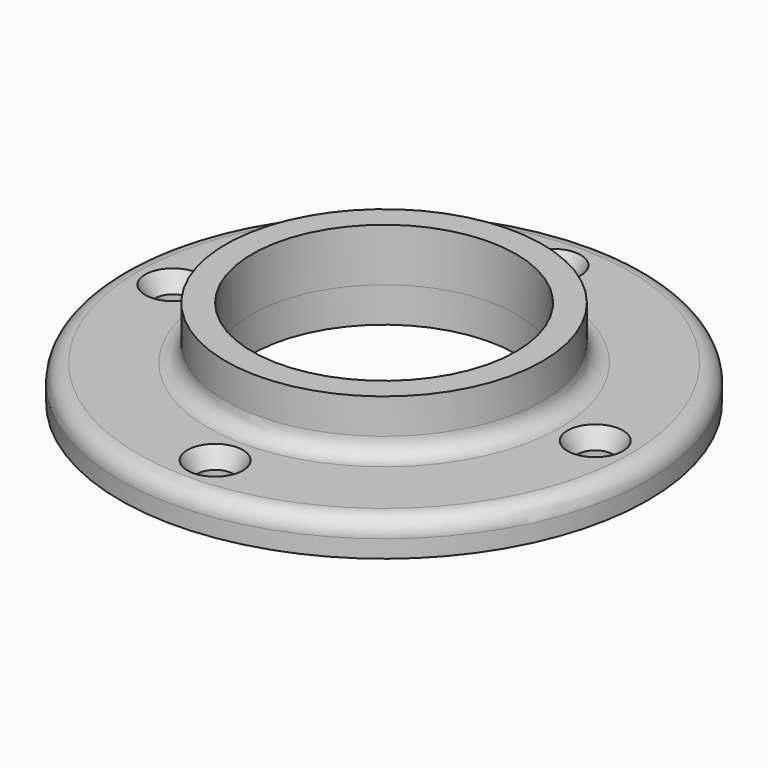
from build123d import *

# Parameters (mm, degrees)
F0_R          = 15
F1_DEPTH      = 1
F1_DEPTH_BACK = 1
F2_R          = 1
F3_DEPTH      = 2
F3_DEPTH_BACK = 2
F3_TAPER_BACK = -30
F4_R          = 9
F4_R_2        = 7.5
F5_DEPTH      = 3
F6_DEPTH      = 5
F7_R          = 0.99999


# Not quite as in the source:
# - a fillet or chamfer is up to 0.001 mm smaller than in the source, because OpenCascade refuses the exact size


with BuildPart() as f1:
    # F0 (on Top) → F1 (new body, two sides)
    with BuildSketch(Plane.XY) as f1_sk:
        Circle(F0_R)
    extrude(amount=F1_DEPTH)
    extrude(f1_sk.sketch, amount=-F1_DEPTH_BACK)

    # F2 (on Top) → F3 (cut, two sides)
    with BuildSketch(Plane.XY) as f3_sk:
        with Locations((12, 0)):
            Circle(F2_R)
        with Locations((0, 12)):
            Circle(F2_R)
        with Locations((-12, 0)):
            Circle(F2_R)
        with Locations((0, -12)):
            Circle(F2_R)
    extrude(amount=-F3_DEPTH, mode=Mode.SUBTRACT)
    extrude(f3_sk.sketch, amount=F3_DEPTH_BACK, taper=F3_TAPER_BACK, mode=Mode.SUBTRACT)

    # F4 (on face) → F5 (join)
    with BuildSketch(Plane.XY.offset(1)):
        Circle(F4_R)
        Circle(F4_R_2, mode=Mode.SUBTRACT)
    extrude(amount=F5_DEPTH)

    # F6 (cut): a face of the model
    f6_faces = [f1.faces().sort_by_distance(p)[0] for p in [
        (0, 0, 1),
    ]]
    extrude(f6_faces, amount=-F6_DEPTH, mode=Mode.SUBTRACT)

    # F7 (radius 1 in the source; OpenCascade refuses exactly that, so slightly less here)
    f7_edges = [f1.edges().sort_by_distance(p)[0] for p in [
        (-15, 0, 1),
        (-9, 0, 1),
    ]]
    fillet(f7_edges, radius=F7_R)


solid = f1.part
